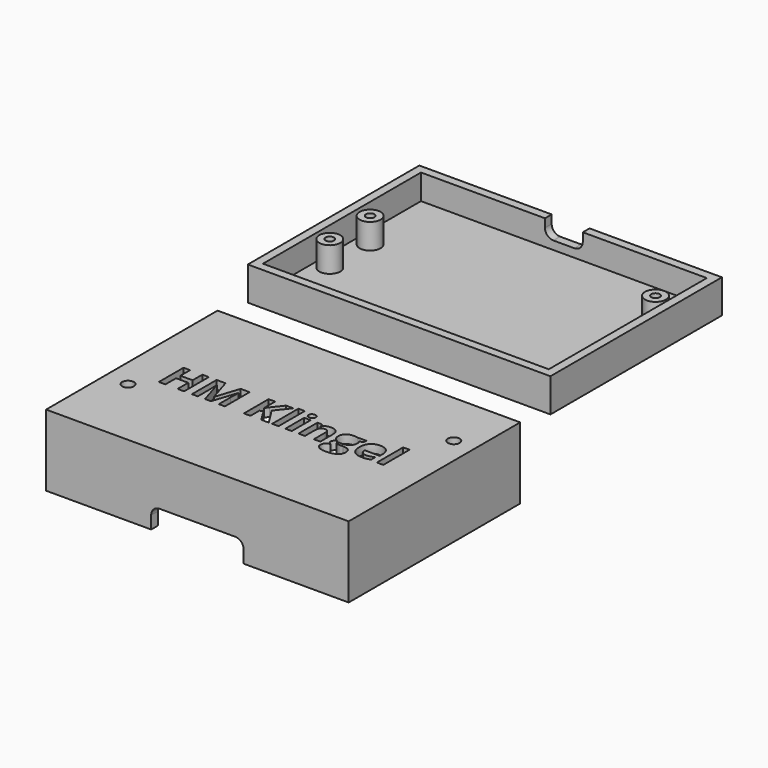
from build123d import *

# Parameters (mm, degrees)
F0_W             = 72
F0_H             = 51
F0_W_2           = 68
F0_H_2           = 47
F0_R             = 2.5
F1_DEPTH         = 2
F3_W             = 72
F3_H             = 51
F3_W_2           = 68
F3_H_2           = 47
F4_DEPTH         = 17
F5_D             = 3
F5_DEPTH         = 3
F5_TIP           = 0.9012909285
F6_W             = 22
F6_H             = 2
F7_DEPTH         = 5
F8_R             = 2
F9_TEXT_SIZE     = 10.2860816458
F10_DEPTH        = 2
F11_DEPTH        = 6
F3_R             = 2.5
F12_DEPTH        = 15
F13_D            = 2.8
F13_DEPTH        = 20
F13_TIP          = 0.8412048666
F17_D            = 2
F17_DEPTH        = 4
F17_TIP          = 0.600860619
F17_ON_F15_D     = 2
F17_ON_F15_DEPTH = 4
F17_ON_F15_TIP   = 0.600860619
F17_ON_F16_D     = 2
F17_ON_F16_DEPTH = 4
F17_ON_F16_TIP   = 0.600860619
F18_W            = 9
F18_H            = 2
F19_DEPTH        = 4
F20_R            = 2
F21_DEPTH        = 2


# Not quite as in the source:
# - Text() gives the source's letters only with a copy of the font that has no kerning and outlines rounded to 1/6400 em; it was checked with that copy


with BuildPart() as f1:
    # F0 (on Top) → F1 (new body)
    with BuildSketch(Plane.XY):
        with Locations((-11.2318283021, -5.1205969751)):
            Rectangle(F0_W, F0_H)
        with Locations((-11.2318283021, -5.1205969751)):
            Rectangle(F0_W_2, F0_H_2, mode=Mode.SUBTRACT)
        with Locations((-11.2318283021, -5.1205969751)):
            Rectangle(F0_W_2, F0_H_2)
        with Locations((-41.7318283021, -13.1205969751)):
            Circle(F0_R, mode=Mode.SUBTRACT)
        with Locations((-41.7318283021, -1.1205969751)):
            Circle(F0_R, mode=Mode.SUBTRACT)
        with Locations((19.7681716979, 6.8794030249)):
            Circle(F0_R, mode=Mode.SUBTRACT)
        with Locations((-41.7318283021, -1.1205969751)):
            Circle(F0_R)
        with Locations((19.7681716979, 6.8794030249)):
            Circle(F0_R)
        with Locations((-41.7318283021, -13.1205969751)):
            Circle(F0_R)
    extrude(amount=-F1_DEPTH)


with BuildPart() as f2_1:
    # F2: copy of F1
    add(f1.part.moved(Location((0, -60, 0))))

    # F3 (on face) → F4 (join)
    with BuildSketch(Plane.XY):
        with Locations((-11.2318283021, -65.1205969751)):
            Rectangle(F3_W, F3_H)
        with Locations((-11.2318283021, -65.1205969751)):
            Rectangle(F3_W_2, F3_H_2, mode=Mode.SUBTRACT)
    extrude(amount=-F4_DEPTH)

    # F5
    with Locations(Plane.XY):
        with Locations((19.7681716979, -53.1205969751), (-41.7318283021, -73.1205969751)):
            Hole(F5_D / 2, depth=F5_DEPTH)
            with Locations((0, 0, -(F5_DEPTH + F5_TIP / 2))):  # 118° drill point
                Cone(0, F5_D / 2, F5_TIP, mode=Mode.SUBTRACT)

    # F6 (on face) → F7 (cut)
    with BuildSketch(Plane(origin=(0, 0, -17), x_dir=(1, 0, 0), z_dir=(0, 0, -1))):
        with Locations((-11.2318283021, 89.6205969751)):
            Rectangle(F6_W, F6_H)
    extrude(amount=-F7_DEPTH, mode=Mode.SUBTRACT)

    # F8
    f8_edges = [f2_1.edges().sort_by_distance(p)[0] for p in [
        (-22.231828, -89.620597, -12),
        (-0.231828, -89.620597, -12),
    ]]
    fillet(f8_edges, radius=F8_R)

    # F9 (on face) → F10 (cut)
    with BuildSketch(Plane.XY):
        with Locations((-38.7318283021, -68.8677521422)):
            Text('HM Klingel', F9_TEXT_SIZE, font='Open Sans', font_style=FontStyle.BOLD, text_align=(TextAlign.LEFT, TextAlign.BOTTOM))
    extrude(amount=-F10_DEPTH, mode=Mode.SUBTRACT)

    # F3 (on face) → F12 (join)
    with BuildSketch(Plane.XY):
        with Locations((19.7681716979, -53.1205969751)):
            Circle(F3_R)
        with Locations((-41.7318283021, -73.1205969751)):
            Circle(F3_R)
    extrude(amount=-F12_DEPTH)

    # F13
    with Locations(Plane.XY):
        with Locations((-41.7318283021, -73.1205969751), (19.7681716979, -53.1205969751)):
            Hole(F13_D / 2, depth=F13_DEPTH)
            with Locations((0, 0, -(F13_DEPTH + F13_TIP / 2))):  # 118° drill point
                Cone(0, F13_D / 2, F13_TIP, mode=Mode.SUBTRACT)

    # F9 (on face) → F21 (cut)
    with BuildSketch(Plane.XY):
        with BuildLine():
            add(Edge.make_bspline(
                [(3.0176091778, -69.1369581853), (2.7339383324, -69.335447417), (2.7339383324, -69.6617090692)],
                knots=[0, 0, 0, 1, 1, 1], degree=2))
            add(Edge.make_bspline(
                [(2.7339383324, -69.6617090692), (2.7339383324, -69.9783275199), (3.037699181, -70.1591375488)],
                knots=[0, 0, 0, 1, 1, 1], degree=2))
            add(Edge.make_bspline(
                [(3.037699181, -70.1591375488), (3.3414600296, -70.3399475778), (3.8895153173, -70.3399475778)],
                knots=[0, 0, 0, 1, 1, 1], degree=2))
            add(Edge.make_bspline(
                [(3.8895153173, -70.3399475778), (4.7124018489, -70.3399475778), (5.1792935236, -70.1133323415)],
                knots=[0, 0, 0, 1, 1, 1], degree=2))
            add(Edge.make_bspline(
                [(5.1792935236, -70.1133323415), (5.6461851983, -69.8867171052), (5.6461851983, -69.4961674428)],
                knots=[0, 0, 0, 1, 1, 1], degree=2))
            add(Edge.make_bspline(
                [(5.6461851983, -69.4961674428), (5.6461851983, -69.1795489921), (5.3705503542, -69.0590089728)],
                knots=[0, 0, 0, 1, 1, 1], degree=2))
            add(Edge.make_bspline(
                [(5.3705503542, -69.0590089728), (5.0949155101, -68.9384689535), (4.5163234176, -68.9384689535)],
                knots=[0, 0, 0, 1, 1, 1], degree=2))
            Line((4.5163234176, -68.9384689535), (3.7223664905, -68.9384689535))
            add(Edge.make_bspline(
                [(3.7223664905, -68.9384689535), (3.3012800232, -68.9384689535), (3.0176091778, -69.1369581853)],
                knots=[0, 0, 0, 1, 1, 1], degree=2))
        make_face()
        with BuildLine():
            add(Edge.make_bspline(
                [(4.1354169566, -64.0766881756), (3.2916368216, -64.0766881756), (3.2916368216, -65.0908315379)],
                knots=[0, 0, 0, 1, 1, 1], degree=2))
            add(Edge.make_bspline(
                [(3.2916368216, -65.0908315379), (3.2916368216, -65.5472764109), (3.4997692549, -65.8140716536)],
                knots=[0, 0, 0, 1, 1, 1], degree=2))
            add(Edge.make_bspline(
                [(3.4997692549, -65.8140716536), (3.7079016882, -66.0808668963), (4.1354169566, -66.0808668963)],
                knots=[0, 0, 0, 1, 1, 1], degree=2))
            add(Edge.make_bspline(
                [(4.1354169566, -66.0808668963), (4.5661466255, -66.0808668963), (4.7670466577, -65.8140716536)],
                knots=[0, 0, 0, 1, 1, 1], degree=2))
            add(Edge.make_bspline(
                [(4.7670466577, -65.8140716536), (4.9679466898, -65.5472764109), (4.9679466898, -65.0908315379)],
                knots=[0, 0, 0, 1, 1, 1], degree=2))
            add(Edge.make_bspline(
                [(4.9679466898, -65.0908315379), (4.9679466898, -64.0766881756), (4.1354169566, -64.0766881756)],
                knots=[0, 0, 0, 1, 1, 1], degree=2))
        make_face()
        with BuildLine():
            add(Edge.make_bspline(
                [(11.0913796696, -64.5459906507), (10.8052980238, -64.2374082014), (10.3183163459, -64.2374082014)],
                knots=[0, 0, 0, 1, 1, 1], degree=2))
            add(Edge.make_bspline(
                [(10.3183163459, -64.2374082014), (9.831334668, -64.2374082014), (9.5548962237, -64.5459906507)],
                knots=[0, 0, 0, 1, 1, 1], degree=2))
            add(Edge.make_bspline(
                [(9.5548962237, -64.5459906507), (9.2784577795, -64.8545731001), (9.2382777731, -65.4219147909)],
                knots=[0, 0, 0, 1, 1, 1], degree=2))
            Line((9.2382777731, -65.4219147909), (11.3887117171, -65.4219147909))
            add(Edge.make_bspline(
                [(11.3887117171, -65.4219147909), (11.3774613153, -64.8545731001), (11.0913796696, -64.5459906507)],
                knots=[0, 0, 0, 1, 1, 1], degree=2))
        make_face()
    extrude(amount=-F21_DEPTH, mode=Mode.SUBTRACT)


with BuildPart() as f1_1:
    add(f1.part)

    # F0 (on Top) → F11 (join)
    with BuildSketch(Plane.XY):
        with Locations((-11.2318283021, -5.1205969751)):
            Rectangle(F0_W, F0_H)
        with Locations((-11.2318283021, -5.1205969751)):
            Rectangle(F0_W_2, F0_H_2, mode=Mode.SUBTRACT)
        with Locations((-41.7318283021, -1.1205969751)):
            Circle(F0_R)
        with Locations((-41.7318283021, -13.1205969751)):
            Circle(F0_R)
        with Locations((19.7681716979, 6.8794030249)):
            Circle(F0_R)
    extrude(amount=F11_DEPTH)

    # F17
    with Locations(Plane.XY.offset(6)):
        with Locations((-41.7318283021, -1.1205969751)):
            Hole(F17_D / 2, depth=F17_DEPTH)
            with Locations((0, 0, -(F17_DEPTH + F17_TIP / 2))):  # 118° drill point
                Cone(0, F17_D / 2, F17_TIP, mode=Mode.SUBTRACT)

    # F17 on F15
    with Locations(Plane.XY.offset(6)):
        with Locations((-41.7318283021, -13.1205969751)):
            Hole(F17_ON_F15_D / 2, depth=F17_ON_F15_DEPTH)
            with Locations((0, 0, -(F17_ON_F15_DEPTH + F17_ON_F15_TIP / 2))):  # 118° drill point
                Cone(0, F17_ON_F15_D / 2, F17_ON_F15_TIP, mode=Mode.SUBTRACT)

    # F17 on F16
    with Locations(Plane.XY.offset(6)):
        with Locations((19.7681716979, 6.8794030249)):
            Hole(F17_ON_F16_D / 2, depth=F17_ON_F16_DEPTH)
            with Locations((0, 0, -(F17_ON_F16_DEPTH + F17_ON_F16_TIP / 2))):  # 118° drill point
                Cone(0, F17_ON_F16_D / 2, F17_ON_F16_TIP, mode=Mode.SUBTRACT)

    # F18 (on face) → F19 (cut)
    with BuildSketch(Plane.XY.offset(6)):
        with Locations((-11.2318283021, 19.3794030249)):
            Rectangle(F18_W, F18_H)
    extrude(amount=-F19_DEPTH, mode=Mode.SUBTRACT)

    # F20
    f20_edges = [f1_1.edges().sort_by_distance(p)[0] for p in [
        (-6.731828, 19.379403, 2),
        (-15.731828, 19.379403, 2),
    ]]
    fillet(f20_edges, radius=F20_R)


solid = Compound([f2_1.part, f1_1.part])
